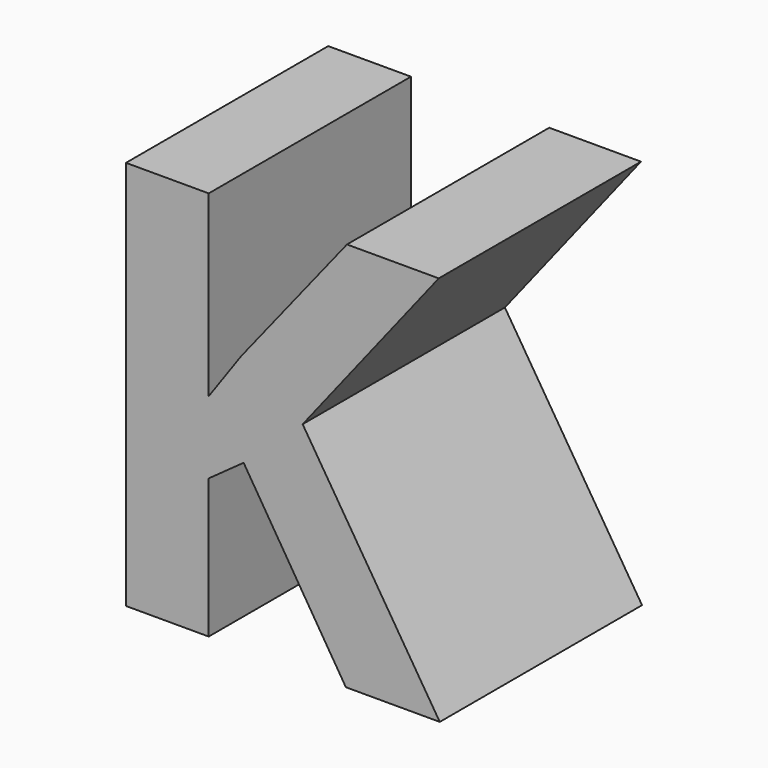
from build123d import *

# Parameters (mm, degrees)
F0_TEXT_SIZE = 54.9074469341
F1_DEPTH     = 12.7


# Not quite as in the source:
# - Text() gives the source's letters only with a copy of the font that has no kerning and outlines rounded to 1/6400 em; it was checked with that copy


with BuildPart() as f1:
    # F0 (on Front) → F1 (new body, symmetric)
    with BuildSketch(Plane.XZ):
        with Locations((0, 0)):
            Text('K', F0_TEXT_SIZE, font='Open Sans', font_style=FontStyle.BOLD, text_align=(TextAlign.LEFT, TextAlign.BOTTOM))
    extrude(amount=F1_DEPTH, both=True)


solid = f1.part
